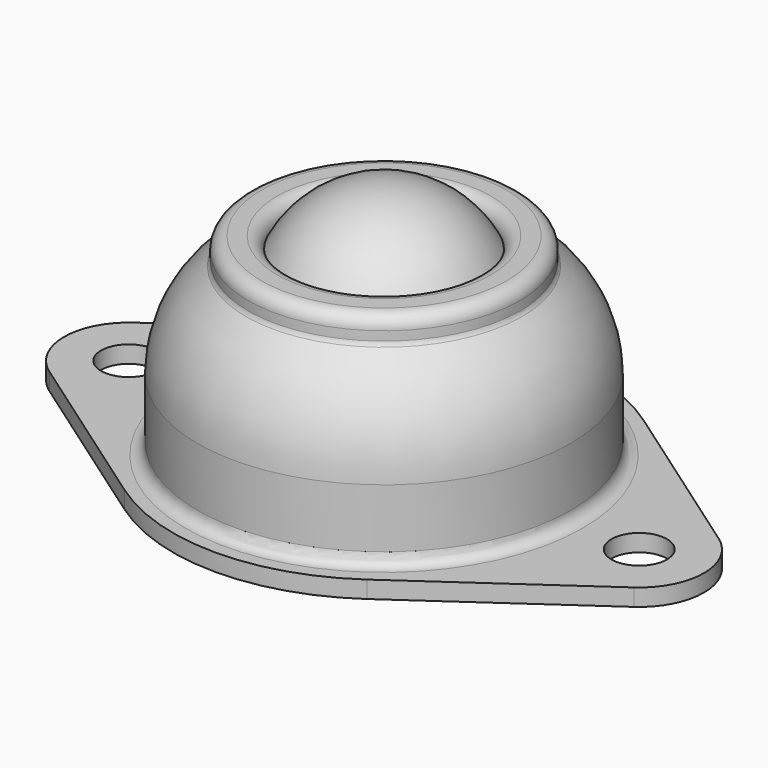
from build123d import *

# Parameters (mm, degrees)
F0_R     = 2.1
F0_R_2   = 14.15
F0_R_3   = 10.3
F0_R_4   = 7.1
F1_DEPTH = 1.3
F2_DEPTH = 14.05
F3_DEPTH = 15.95
F4_R     = 0.9
F6_R     = 0.4
F7_R     = 1


# Not quite as in the source:
# - a fillet or chamfer that OpenCascade refuses, or shapes differently, is made with other operations: its cross-section is extruded or revolved along the edge and cut away or added


with BuildPart() as f1:
    # F0 (on Top) → F1 (new body)
    with BuildSketch(Plane.XY):
        with BuildLine():
            Line((9.1782945736, -13.1056823065), (22.1608527132, -4.0136152064))
            ThreePointArc((22.1608527132, -4.0136152064), (24.25, 0), (22.1608527132, 4.0136152064))
            Line((22.1608527132, 4.0136152064), (9.1782945736, 13.1056823065))
            ThreePointArc((9.1782945736, 13.1056823065), (0, 16), (-9.1782945736, 13.1056823065))
            Line((-9.1782945736, 13.1056823065), (-22.1608527132, 4.0136152064))
            ThreePointArc((-22.1608527132, 4.0136152064), (-24.25, 0), (-22.1608527132, -4.0136152064))
            Line((-22.1608527132, -4.0136152064), (-9.1782945736, -13.1056823065))
            ThreePointArc((-9.1782945736, -13.1056823065), (0, -16), (9.1782945736, -13.1056823065))
        make_face()
        with Locations((-19.35, 0)):
            Circle(F0_R, mode=Mode.SUBTRACT)
        Circle(F0_R_2, mode=Mode.SUBTRACT)
        with Locations((19.35, 0)):
            Circle(F0_R, mode=Mode.SUBTRACT)
        Circle(F0_R_2)
        Circle(F0_R_3, mode=Mode.SUBTRACT)
        Circle(F0_R_3)
        Circle(F0_R_4, mode=Mode.SUBTRACT)
        Circle(F0_R_4)
    extrude(amount=F1_DEPTH)

    # F0 (on Top) → F2 (join)
    with BuildSketch(Plane.XY):
        Circle(F0_R_2)
        Circle(F0_R_3, mode=Mode.SUBTRACT)
        Circle(F0_R_3)
        Circle(F0_R_4, mode=Mode.SUBTRACT)
        Circle(F0_R_4)
    extrude(amount=F2_DEPTH)

    # F0 (on Top) → F3 (join)
    with BuildSketch(Plane.XY):
        Circle(F0_R_3)
        Circle(F0_R_4, mode=Mode.SUBTRACT)
    extrude(amount=F3_DEPTH)

    # F4
    f4_edges = [f1.edges().sort_by_distance(p)[0] for p in [
        (-14.15, 0, 1.3),
    ]]
    fillet(f4_edges, radius=F4_R)

    # F5: fillet of radius 9 on 1 edges, made by hand

    # F5_s1 → F5_t2 (revolve, cut)
    with BuildSketch(Plane.XZ):
        with BuildLine():
            ThreePointArc((14.15, 6.6691125195), (13.129661647, 10.8314435971), (10.3, 14.05))
            Line((10.3, 14.05), (14.15, 14.05))
            Line((14.15, 14.05), (14.15, 6.6691125195))
        make_face()
    revolve(axis=Axis((0, 0, 14.05), (0, 0, 1)), mode=Mode.SUBTRACT)

    # F6
    f6_edges = [f1.edges().sort_by_distance(p)[0] for p in [
        (-10.3, 0, 14.05),
    ]]
    fillet(f6_edges, radius=F6_R)

    # F7
    f7_edges = [f1.edges().sort_by_distance(p)[0] for p in [
        (-10.3, 0, 15.95),
        (-7.1, 0, 15.95),
    ]]
    fillet(f7_edges, radius=F7_R)

    # F9 (on offset) → F10 (revolve)
    with BuildSketch(Plane.XY.offset(11.35)):
        with BuildLine():
            Line((0, -8), (0, 8))
            ThreePointArc((0, 8), (-8, 0), (0, -8))
        make_face()
    revolve(axis=Axis((0, -0.0622457136, 11.35), (0, 1, 0)))


solid = f1.part
